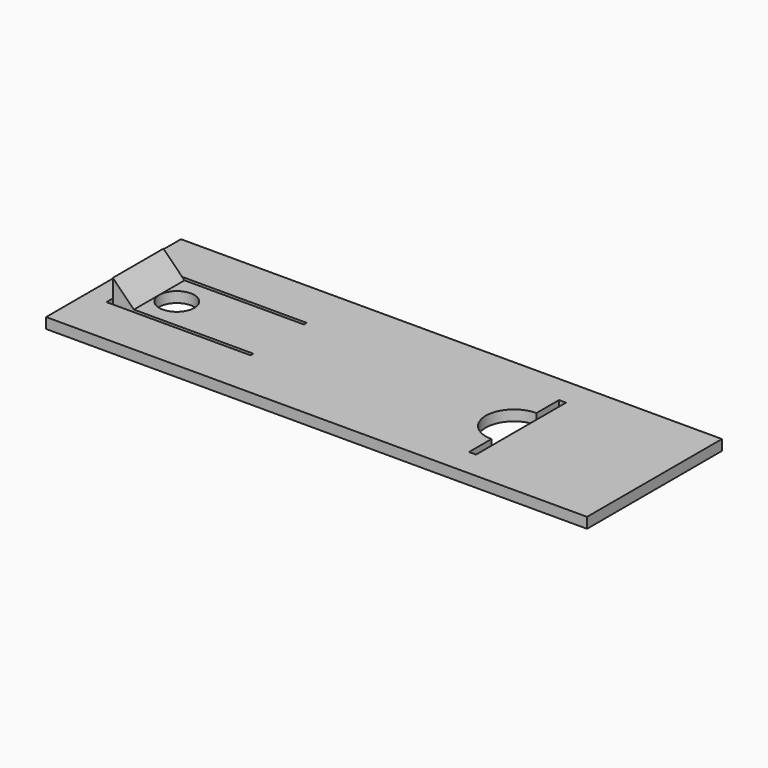
from build123d import *

# Parameters (mm, degrees)
F0_W     = 77
F0_H     = 24
F0_R     = 2.5
F1_DEPTH = 1.5
F2_W     = 3
F2_H     = 9
F3_DEPTH = 3
F4_SIZE  = 2.99999


# Not quite as in the source:
# - a fillet or chamfer is up to 0.001 mm smaller than in the source, because OpenCascade refuses the exact size


with BuildPart() as f1:
    # F0 (on Top) → F1 (new body)
    with BuildSketch(Plane.XY):
        Rectangle(F0_W, F0_H)
        with Locations((-29.5, 0)):
            Circle(F0_R, mode=Mode.SUBTRACT)
        Polygon((-35.5, -5), (-35.5, 5), (-15, 5), (-15, 4.5), (-35, 4.5), (-35, -4.5), (-15, -4.5), (-15, -5), align=None, mode=Mode.SUBTRACT)
        with BuildLine():
            Line((18.5, 4), (18.5, 8))
            Line((18.5, 8), (19.5, 8))
            Line((19.5, 8), (19.5, -8))
            Line((19.5, -8), (18.5, -8))
            Line((18.5, -8), (18.5, -4))
            ThreePointArc((18.5, -4), (14.5, 0), (18.5, 4))
        make_face(mode=Mode.SUBTRACT)
    extrude(amount=F1_DEPTH)

    # F2 (on face) → F3 (join)
    with BuildSketch(Plane.XY.offset(1.5)):
        with Locations((-33.5, 0)):
            Rectangle(F2_W, F2_H)
    extrude(amount=F3_DEPTH)

    # F4 (size 3 in the source; OpenCascade refuses exactly that, so slightly less here)
    f4_edges = [f1.edges().sort_by_distance(p)[0] for p in [
        (-32, 0, 4.5),
    ]]
    chamfer(f4_edges, length=F4_SIZE)


solid = f1.part
